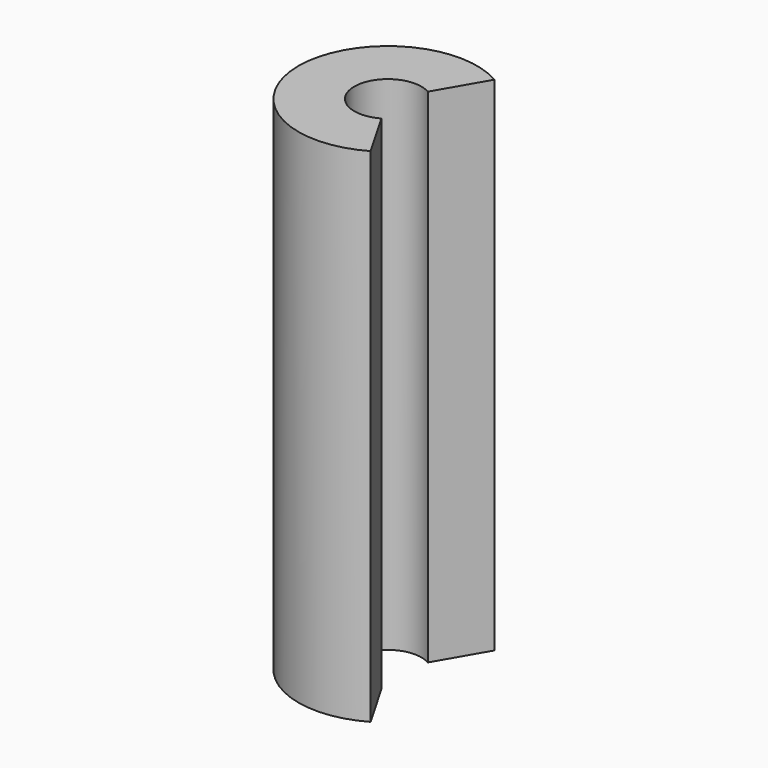
from build123d import *

# Parameters (mm, degrees)
F0_W          = 20.32
F0_H          = 114.3
F1_ANGLE_BACK = 120
F1_ANGLE      = 240
F2_W          = 7.62
F2_H          = 127


with BuildPart() as f1:
    # F0 (on Front) → F1 (revolve)
    with BuildSketch(Plane.XZ, mode=Mode.PRIVATE) as f1_sk:
        with Locations((-10.16, -11.4712095437)):
            Rectangle(F0_W, F0_H)
    revolve(f1_sk.sketch.rotate(Axis((0, 0, -11.4712095437), (0, 0, -1)), -F1_ANGLE_BACK), axis=Axis((0, 0, -11.4712095437), (0, 0, -1)), revolution_arc=F1_ANGLE)

    # F2 (on Front) → F3 (revolve, cut)
    with BuildSketch(Plane.XZ):
        with Locations((-3.81, -5.3986597389)):
            Rectangle(F2_W, F2_H)
    revolve(axis=Axis((0, 0, -5.3986597389), (0, 0, -1)), mode=Mode.SUBTRACT)


solid = f1.part
